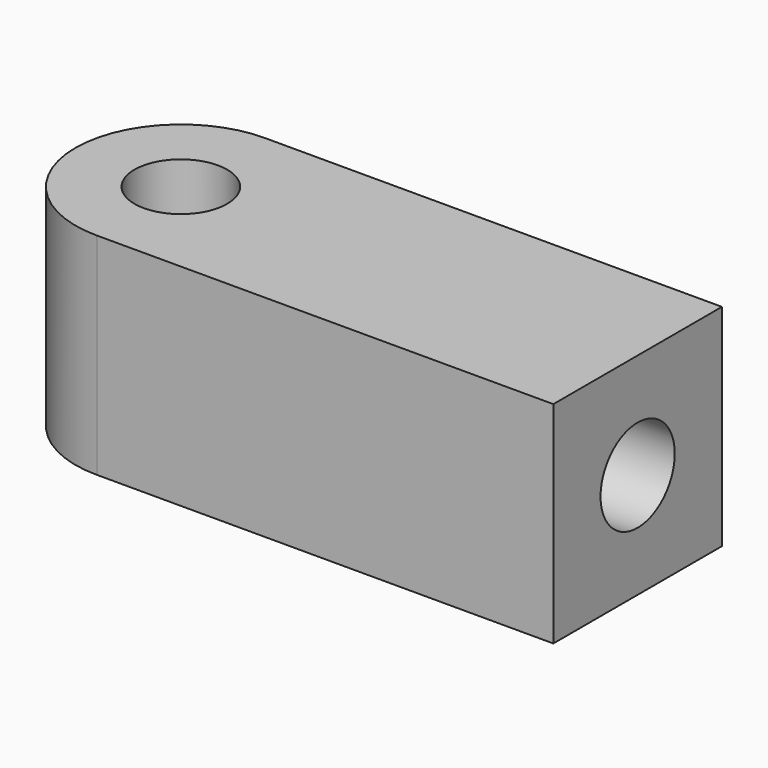
from build123d import *

# Parameters (mm, degrees)
F1_DEPTH       = 15
F3_DEPTH       = 15
F5_D           = 13.2
F5_DEPTH       = 60
F5_CBORE_D     = 19.25
F5_CBORE_DEPTH = 0
F5_TIP         = 3.9656800856
F7_D           = 13.2
F7_DEPTH       = 60
F7_CBORE_D     = 19.25
F7_CBORE_DEPTH = 0
F7_TIP         = 3.9656800856


# Not quite as in the source:
# - ends of sketch curves that miss each other by under 0.0002 mm in the source are joined


with BuildPart() as f1:
    # F0 (on Top) → F1 (new body, symmetric)
    with BuildSketch(Plane.XY):
        with BuildLine():
            Line((-32.5, -15), (-32.5, 15))
            ThreePointArc((-32.5, 15), (-47.5306145724, 0), (-32.5, -15))
        make_face()
        with BuildLine():
            ThreePointArc((-32.5000000638, -14.9999687584), (-21.9131945085, -10.595772326), (-17.5306145724, 0))
            ThreePointArc((-17.5306145724, 0), (-21.9131945085, 10.595772326), (-32.5000000638, 14.9999687584))
            Line((-32.5000000638, 14.9999687584), (-32.5000000638, -14.9999687584))
        make_face()
        with BuildLine():
            ThreePointArc((-32.5000000638, 14.9999687584), (-21.9131945085, 10.595772326), (-17.5306145724, 0))
            ThreePointArc((-17.5306145724, 0), (-21.9131945085, -10.595772326), (-32.5000000638, -14.9999687584))
            Line((-32.5000000638, -14.9999687584), (32.5, -15))
            Line((32.5, -15), (32.5, 15))
            Line((32.5, 15), (-32.5000000638, 14.9999687584))
        make_face()
    extrude(amount=F1_DEPTH, both=True)

    # F2 (on Right) → F3 (cut)
    with BuildSketch(Plane.YZ):
        Polygon((9.5593853593, 5.4426588685), (9.4931735239, -5.5573411315), (-0.0662118354, -11), (17.534378916, -11.1163873225), (17.534378916, 11), (0.0662118354, 11), align=None)
        Polygon((-0.0662118354, -11), (9.4931735239, -5.5573411315), (9.5593853593, 5.4426588685), (0.0662118354, 11), (-9.4931735239, 5.5573411315), (-9.5593853593, -5.4426588685), align=None)
    extrude(amount=-F3_DEPTH, mode=Mode.SUBTRACT)

    # F5
    with Locations(Plane(origin=(0, 0, -15), x_dir=(1, 0, 0), z_dir=(0, 0, -1))):
        with Locations((-32.5306145724, 0)):
            CounterBoreHole(F5_D / 2, F5_CBORE_D / 2, F5_CBORE_DEPTH, depth=F5_DEPTH)
            with Locations((0, 0, -(F5_DEPTH + F5_TIP / 2))):  # 118° drill point
                Cone(0, F5_D / 2, F5_TIP, mode=Mode.SUBTRACT)

    # F7
    with Locations(Plane.YZ.offset(32.5)):
        with Locations((0, 0)):
            CounterBoreHole(F7_D / 2, F7_CBORE_D / 2, F7_CBORE_DEPTH, depth=F7_DEPTH)
            with Locations((0, 0, -(F7_DEPTH + F7_TIP / 2))):  # 118° drill point
                Cone(0, F7_D / 2, F7_TIP, mode=Mode.SUBTRACT)


solid = f1.part
